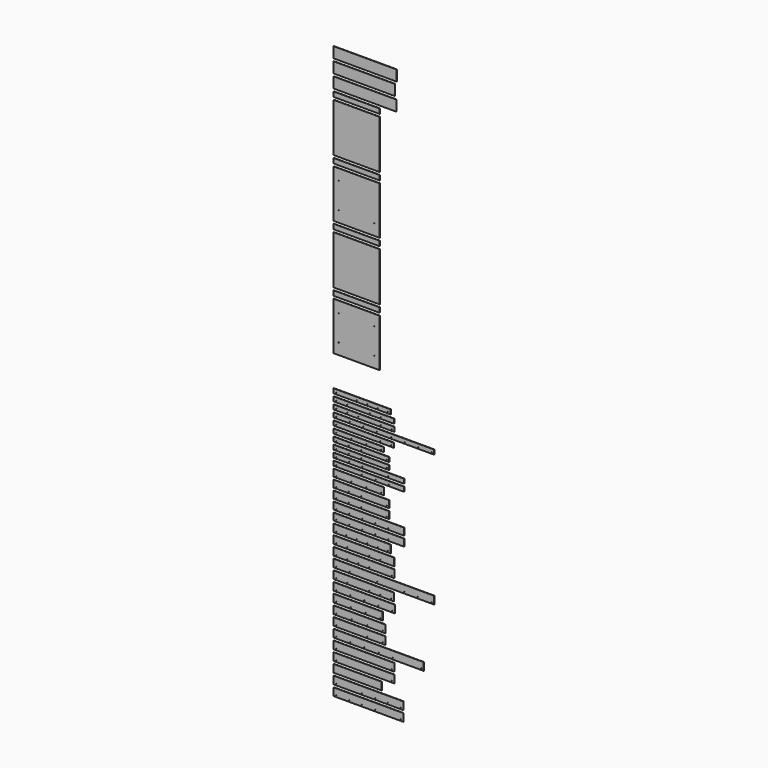
from build123d import *

# Parameters (mm, degrees)
F0_W     = 621.50625
F0_H     = 105.56875
F1_DEPTH = 3.175
F0_W_2   = 604.8375
F0_W_3   = 618.33125
F0_W_4   = 454.025
F0_H_2   = 47.625
F0_H_3   = 479.425
F0_H_4   = 473.075
F0_R     = 2.38125
F0_W_5   = 561.975
F0_H_5   = 76.2
F0_W_6   = 596.9
F0_W_7   = 598.4875
F0_W_8   = 992.1875
F0_W_9   = 595.3125
F0_W_10  = 484.1875
F0_W_11  = 511.175
F0_W_12  = 889
F0_W_13  = 600.075
F0_W_14  = 473.075
F0_W_15  = 688.975
F0_R_2   = 2.159
F0_H_6   = 44.45
F0_W_16  = 495.3
F0_W_17  = 547.6875
F0_W_18  = 695.325
F0_H_7   = 69.85


# Not quite as in the source:
# - a feature names something its author has since deleted; it is built from what else it names


with BuildPart() as f1:
    # F0 (on Front) → F1 (new body)
    with BuildSketch(Plane.XZ):
        with Locations((310.753125, -78.184375)):
            Rectangle(F0_W, F0_H)
    extrude(amount=F1_DEPTH)


with BuildPart() as f1b:
    # F0 (on Front) → F1, piece 2 (new body)
    with BuildSketch(Plane.XZ):
        with Locations((302.41875, -209.153125)):
            Rectangle(F0_W_2, F0_H)
    extrude(amount=F1_DEPTH)


with BuildPart() as f1c:
    # F0 (on Front) → F1, piece 3 (new body)
    with BuildSketch(Plane.XZ):
        with Locations((309.165625, -340.121875)):
            Rectangle(F0_W_3, F0_H)
    extrude(amount=F1_DEPTH)


with BuildPart() as f1d:
    # F0 (on Front) → F1, piece 4 (new body)
    with BuildSketch(Plane.XZ):
        with Locations((227.0125, -442.11875)):
            Rectangle(F0_W_4, F0_H_2)
    extrude(amount=F1_DEPTH)


with BuildPart() as f1e:
    # F0 (on Front) → F1, piece 5 (new body)
    with BuildSketch(Plane.XZ):
        with Locations((227.0125, -731.04375)):
            Rectangle(F0_W_4, F0_H_3)
    extrude(amount=F1_DEPTH)


with BuildPart() as f1f:
    # F0 (on Front) → F1, piece 6 (new body)
    with BuildSketch(Plane.XZ):
        with Locations((227.0125, -1019.96875)):
            Rectangle(F0_W_4, F0_H_2)
    extrude(amount=F1_DEPTH)


with BuildPart() as f1g:
    # F0 (on Front) → F1, piece 7 (new body)
    with BuildSketch(Plane.XZ):
        with Locations((227.0125, -1305.71875)):
            Rectangle(F0_W_4, F0_H_4)
        with Locations((50.8, -1432.71875)):
            Circle(F0_R, mode=Mode.SUBTRACT)
        with Locations((50.8, -1178.71875)):
            Circle(F0_R, mode=Mode.SUBTRACT)
        with Locations((403.225, -1432.71875)):
            Circle(F0_R, mode=Mode.SUBTRACT)
        with Locations((403.225, -1178.71875)):
            Circle(F0_R, mode=Mode.SUBTRACT)
    extrude(amount=F1_DEPTH)


with BuildPart() as f1h:
    # F0 (on Front) → F1, piece 8 (new body)
    with BuildSketch(Plane.XZ):
        with Locations((227.0125, -1591.46875)):
            Rectangle(F0_W_4, F0_H_2)
    extrude(amount=F1_DEPTH)


with BuildPart() as f1i:
    # F0 (on Front) → F1, piece 9 (new body)
    with BuildSketch(Plane.XZ):
        with Locations((227.0125, -1880.39375)):
            Rectangle(F0_W_4, F0_H_3)
    extrude(amount=F1_DEPTH)


with BuildPart() as f1j:
    # F0 (on Front) → F1, piece 10 (new body)
    with BuildSketch(Plane.XZ):
        with Locations((227.0125, -2169.31875)):
            Rectangle(F0_W_4, F0_H_2)
    extrude(amount=F1_DEPTH)


with BuildPart() as f1k:
    # F0 (on Front) → F1, piece 11 (new body)
    with BuildSketch(Plane.XZ):
        with Locations((227.0125, -2455.06875)):
            Rectangle(F0_W_4, F0_H_4)
        with Locations((50.8, -2582.06875)):
            Circle(F0_R, mode=Mode.SUBTRACT)
        with Locations((50.8, -2328.06875)):
            Circle(F0_R, mode=Mode.SUBTRACT)
        with Locations((403.225, -2582.06875)):
            Circle(F0_R, mode=Mode.SUBTRACT)
        with Locations((403.225, -2328.06875)):
            Circle(F0_R, mode=Mode.SUBTRACT)
    extrude(amount=F1_DEPTH)


with BuildPart() as f1l:
    # F0 (on Front) → F1, piece 12 (new body)
    with BuildSketch(Plane.XZ):
        with Locations((280.9875, -4209.25625)):
            Rectangle(F0_W_5, F0_H_5)
        with Locations((25.4, -4233.06875)):
            Circle(F0_R, mode=Mode.SUBTRACT)
        with Locations((127, -4233.06875)):
            Circle(F0_R, mode=Mode.SUBTRACT)
        with Locations((228.6, -4233.06875)):
            Circle(F0_R, mode=Mode.SUBTRACT)
        with Locations((333.375, -4233.06875)):
            Circle(F0_R, mode=Mode.SUBTRACT)
        with Locations((434.975, -4233.06875)):
            Circle(F0_R, mode=Mode.SUBTRACT)
        with Locations((536.575, -4233.06875)):
            Circle(F0_R, mode=Mode.SUBTRACT)
    extrude(amount=F1_DEPTH)


with BuildPart() as f1m:
    # F0 (on Front) → F1, piece 13 (new body)
    with BuildSketch(Plane.XZ):
        with Locations((298.45, -4310.85625)):
            Rectangle(F0_W_6, F0_H_5)
        with Locations((25.4, -4334.66875)):
            Circle(F0_R, mode=Mode.SUBTRACT)
        with Locations((134.9375, -4334.66875)):
            Circle(F0_R, mode=Mode.SUBTRACT)
        with Locations((244.475, -4334.66875)):
            Circle(F0_R, mode=Mode.SUBTRACT)
        with Locations((352.425, -4334.66875)):
            Circle(F0_R, mode=Mode.SUBTRACT)
        with Locations((461.9625, -4334.66875)):
            Circle(F0_R, mode=Mode.SUBTRACT)
        with Locations((571.5, -4334.66875)):
            Circle(F0_R, mode=Mode.SUBTRACT)
    extrude(amount=F1_DEPTH)


with BuildPart() as f1n:
    # F0 (on Front) → F1, piece 14 (new body)
    with BuildSketch(Plane.XZ):
        with Locations((299.24375, -4412.45625)):
            Rectangle(F0_W_7, F0_H_5)
        with Locations((25.4, -4436.26875)):
            Circle(F0_R, mode=Mode.SUBTRACT)
        with Locations((134.9375, -4436.26875)):
            Circle(F0_R, mode=Mode.SUBTRACT)
        with Locations((244.475, -4436.26875)):
            Circle(F0_R, mode=Mode.SUBTRACT)
        with Locations((354.0125, -4436.26875)):
            Circle(F0_R, mode=Mode.SUBTRACT)
        with Locations((463.55, -4436.26875)):
            Circle(F0_R, mode=Mode.SUBTRACT)
        with Locations((573.0875, -4436.26875)):
            Circle(F0_R, mode=Mode.SUBTRACT)
    extrude(amount=F1_DEPTH)


with BuildPart() as f1o:
    # F0 (on Front) → F1, piece 15 (new body)
    with BuildSketch(Plane.XZ):
        with Locations((496.09375, -4514.05625)):
            Rectangle(F0_W_8, F0_H_5)
        with Locations((25.4, -4537.86875)):
            Circle(F0_R, mode=Mode.SUBTRACT)
        with Locations((160.3375, -4537.86875)):
            Circle(F0_R, mode=Mode.SUBTRACT)
        with Locations((295.275, -4537.86875)):
            Circle(F0_R, mode=Mode.SUBTRACT)
        with Locations((430.2125, -4537.86875)):
            Circle(F0_R, mode=Mode.SUBTRACT)
        with Locations((561.975, -4537.86875)):
            Circle(F0_R, mode=Mode.SUBTRACT)
        with Locations((696.9125, -4537.86875)):
            Circle(F0_R, mode=Mode.SUBTRACT)
        with Locations((831.85, -4537.86875)):
            Circle(F0_R, mode=Mode.SUBTRACT)
        with Locations((966.7875, -4537.86875)):
            Circle(F0_R, mode=Mode.SUBTRACT)
    extrude(amount=F1_DEPTH)


with BuildPart() as f1p:
    # F0 (on Front) → F1, piece 16 (new body)
    with BuildSketch(Plane.XZ):
        with Locations((297.65625, -4615.65625)):
            Rectangle(F0_W_9, F0_H_5)
        with Locations((25.4, -4639.46875)):
            Circle(F0_R, mode=Mode.SUBTRACT)
        with Locations((133.35, -4639.46875)):
            Circle(F0_R, mode=Mode.SUBTRACT)
        with Locations((241.3, -4639.46875)):
            Circle(F0_R, mode=Mode.SUBTRACT)
        with Locations((354.0125, -4639.46875)):
            Circle(F0_R, mode=Mode.SUBTRACT)
        with Locations((461.9625, -4639.46875)):
            Circle(F0_R, mode=Mode.SUBTRACT)
        with Locations((569.9125, -4639.46875)):
            Circle(F0_R, mode=Mode.SUBTRACT)
    extrude(amount=F1_DEPTH)


with BuildPart() as f1q:
    # F0 (on Front) → F1, piece 17 (new body)
    with BuildSketch(Plane.XZ):
        with Locations((302.41875, -4717.25625)):
            Rectangle(F0_W_2, F0_H_5)
        with Locations((25.4, -4741.06875)):
            Circle(F0_R, mode=Mode.SUBTRACT)
        with Locations((163.5125, -4741.06875)):
            Circle(F0_R, mode=Mode.SUBTRACT)
        with Locations((302.41875, -4741.06875)):
            Circle(F0_R, mode=Mode.SUBTRACT)
        with Locations((441.325, -4741.06875)):
            Circle(F0_R, mode=Mode.SUBTRACT)
        with Locations((579.4375, -4741.06875)):
            Circle(F0_R, mode=Mode.SUBTRACT)
    extrude(amount=F1_DEPTH)


with BuildPart() as f1r:
    # F0 (on Front) → F1, piece 18 (new body)
    with BuildSketch(Plane.XZ):
        with Locations((242.09375, -4818.85625)):
            Rectangle(F0_W_10, F0_H_5)
        with Locations((25.4, -4842.66875)):
            Circle(F0_R, mode=Mode.SUBTRACT)
        with Locations((168.275, -4842.66875)):
            Circle(F0_R, mode=Mode.SUBTRACT)
        with Locations((315.9125, -4842.66875)):
            Circle(F0_R, mode=Mode.SUBTRACT)
        with Locations((458.7875, -4842.66875)):
            Circle(F0_R, mode=Mode.SUBTRACT)
    extrude(amount=F1_DEPTH)


with BuildPart() as f1s:
    # F0 (on Front) → F1, piece 19 (new body)
    with BuildSketch(Plane.XZ):
        with Locations((255.5875, -4920.45625)):
            Rectangle(F0_W_11, F0_H_5)
        with Locations((25.4, -4944.26875)):
            Circle(F0_R, mode=Mode.SUBTRACT)
        with Locations((177.8, -4944.26875)):
            Circle(F0_R, mode=Mode.SUBTRACT)
        with Locations((333.375, -4944.26875)):
            Circle(F0_R, mode=Mode.SUBTRACT)
        with Locations((485.775, -4944.26875)):
            Circle(F0_R, mode=Mode.SUBTRACT)
    extrude(amount=F1_DEPTH)


with BuildPart() as f1t:
    # F0 (on Front) → F1, piece 20 (new body)
    with BuildSketch(Plane.XZ):
        with Locations((255.5875, -5022.05625)):
            Rectangle(F0_W_11, F0_H_5)
        with Locations((25.4, -5045.86875)):
            Circle(F0_R, mode=Mode.SUBTRACT)
        with Locations((177.8, -5045.86875)):
            Circle(F0_R, mode=Mode.SUBTRACT)
        with Locations((333.375, -5045.86875)):
            Circle(F0_R, mode=Mode.SUBTRACT)
        with Locations((485.775, -5045.86875)):
            Circle(F0_R, mode=Mode.SUBTRACT)
    extrude(amount=F1_DEPTH)


with BuildPart() as f1u:
    # F0 (on Front) → F1, piece 21 (new body)
    with BuildSketch(Plane.XZ):
        with Locations((444.5, -5123.65625)):
            Rectangle(F0_W_12, F0_H_5)
        with Locations((25.4, -5147.46875)):
            Circle(F0_R, mode=Mode.SUBTRACT)
        with Locations((165.1, -5147.46875)):
            Circle(F0_R, mode=Mode.SUBTRACT)
        with Locations((304.8, -5147.46875)):
            Circle(F0_R, mode=Mode.SUBTRACT)
        with Locations((444.5, -5147.46875)):
            Circle(F0_R, mode=Mode.SUBTRACT)
        with Locations((584.2, -5147.46875)):
            Circle(F0_R, mode=Mode.SUBTRACT)
        with Locations((723.9, -5147.46875)):
            Circle(F0_R, mode=Mode.SUBTRACT)
        with Locations((863.6, -5147.46875)):
            Circle(F0_R, mode=Mode.SUBTRACT)
    extrude(amount=F1_DEPTH)


with BuildPart() as f1v:
    # F0 (on Front) → F1, piece 22 (new body)
    with BuildSketch(Plane.XZ):
        with Locations((300.0375, -5225.25625)):
            Rectangle(F0_W_13, F0_H_5)
        with Locations((25.4, -5249.06875)):
            Circle(F0_R, mode=Mode.SUBTRACT)
        with Locations((161.925, -5249.06875)):
            Circle(F0_R, mode=Mode.SUBTRACT)
        with Locations((300.0375, -5249.06875)):
            Circle(F0_R, mode=Mode.SUBTRACT)
        with Locations((438.15, -5249.06875)):
            Circle(F0_R, mode=Mode.SUBTRACT)
        with Locations((574.675, -5249.06875)):
            Circle(F0_R, mode=Mode.SUBTRACT)
    extrude(amount=F1_DEPTH)


with BuildPart() as f1w:
    # F0 (on Front) → F1, piece 23 (new body)
    with BuildSketch(Plane.XZ):
        with Locations((300.0375, -5326.85625)):
            Rectangle(F0_W_13, F0_H_5)
        with Locations((25.4, -5350.66875)):
            Circle(F0_R, mode=Mode.SUBTRACT)
        with Locations((161.925, -5350.66875)):
            Circle(F0_R, mode=Mode.SUBTRACT)
        with Locations((300.0375, -5350.66875)):
            Circle(F0_R, mode=Mode.SUBTRACT)
        with Locations((438.15, -5350.66875)):
            Circle(F0_R, mode=Mode.SUBTRACT)
        with Locations((574.675, -5350.66875)):
            Circle(F0_R, mode=Mode.SUBTRACT)
    extrude(amount=F1_DEPTH)


with BuildPart() as f1x:
    # F0 (on Front) → F1, piece 24 (new body)
    with BuildSketch(Plane.XZ):
        with Locations((236.5375, -5428.45625)):
            Rectangle(F0_W_14, F0_H_5)
    extrude(amount=F1_DEPTH)


with BuildPart() as f1y:
    # F0 (on Front) → F1, piece 25 (new body)
    with BuildSketch(Plane.XZ):
        with Locations((344.4875, -5530.05625)):
            Rectangle(F0_W_15, F0_H_5)
        with Locations((25.4, -5553.86875)):
            Circle(F0_R, mode=Mode.SUBTRACT)
        with Locations((152.4, -5553.86875)):
            Circle(F0_R, mode=Mode.SUBTRACT)
        with Locations((279.4, -5553.86875)):
            Circle(F0_R, mode=Mode.SUBTRACT)
        with Locations((409.575, -5553.86875)):
            Circle(F0_R, mode=Mode.SUBTRACT)
        with Locations((536.575, -5553.86875)):
            Circle(F0_R, mode=Mode.SUBTRACT)
        with Locations((663.575, -5553.86875)):
            Circle(F0_R, mode=Mode.SUBTRACT)
    extrude(amount=F1_DEPTH)


with BuildPart() as f1z:
    # F0 (on Front) → F1, piece 26 (new body)
    with BuildSketch(Plane.XZ):
        with Locations((344.4875, -5631.65625)):
            Rectangle(F0_W_15, F0_H_5)
        with Locations((25.4, -5655.46875)):
            Circle(F0_R_2, mode=Mode.SUBTRACT)
        with Locations((152.4, -5655.46875)):
            Circle(F0_R_2, mode=Mode.SUBTRACT)
        with Locations((279.4, -5655.46875)):
            Circle(F0_R_2, mode=Mode.SUBTRACT)
        with Locations((409.575, -5655.46875)):
            Circle(F0_R_2, mode=Mode.SUBTRACT)
        with Locations((536.575, -5655.46875)):
            Circle(F0_R_2, mode=Mode.SUBTRACT)
        with Locations((663.575, -5655.46875)):
            Circle(F0_R_2, mode=Mode.SUBTRACT)
    extrude(amount=F1_DEPTH)


with BuildPart() as f1ba:
    # F0 (on Front) → F1, piece 27 (new body)
    with BuildSketch(Plane.XZ):
        with Locations((280.9875, -3018.63125)):
            Rectangle(F0_W_5, F0_H_6)
        with Locations((25.4, -3026.56875)):
            Circle(F0_R, mode=Mode.SUBTRACT)
        with Locations((127, -3026.56875)):
            Circle(F0_R, mode=Mode.SUBTRACT)
        with Locations((228.6, -3026.56875)):
            Circle(F0_R, mode=Mode.SUBTRACT)
        with Locations((333.375, -3026.56875)):
            Circle(F0_R, mode=Mode.SUBTRACT)
        with Locations((434.975, -3026.56875)):
            Circle(F0_R, mode=Mode.SUBTRACT)
        with Locations((536.575, -3026.56875)):
            Circle(F0_R, mode=Mode.SUBTRACT)
    extrude(amount=F1_DEPTH)


with BuildPart() as f1bb:
    # F0 (on Front) → F1, piece 28 (new body)
    with BuildSketch(Plane.XZ):
        with Locations((298.45, -3088.48125)):
            Rectangle(F0_W_6, F0_H_6)
        with Locations((25.4, -3096.41875)):
            Circle(F0_R, mode=Mode.SUBTRACT)
        with Locations((133.35, -3096.41875)):
            Circle(F0_R, mode=Mode.SUBTRACT)
        with Locations((241.3, -3096.41875)):
            Circle(F0_R, mode=Mode.SUBTRACT)
        with Locations((355.6, -3096.41875)):
            Circle(F0_R, mode=Mode.SUBTRACT)
        with Locations((463.55, -3096.41875)):
            Circle(F0_R, mode=Mode.SUBTRACT)
        with Locations((571.5, -3096.41875)):
            Circle(F0_R, mode=Mode.SUBTRACT)
    extrude(amount=F1_DEPTH)


with BuildPart() as f1bc:
    # F0 (on Front) → F1, piece 29 (new body)
    with BuildSketch(Plane.XZ):
        with Locations((299.24375, -3158.33125)):
            Rectangle(F0_W_7, F0_H_6)
        with Locations((25.4, -3166.26875)):
            Circle(F0_R, mode=Mode.SUBTRACT)
        with Locations((134.9375, -3166.26875)):
            Circle(F0_R, mode=Mode.SUBTRACT)
        with Locations((244.475, -3166.26875)):
            Circle(F0_R, mode=Mode.SUBTRACT)
        with Locations((354.0125, -3166.26875)):
            Circle(F0_R, mode=Mode.SUBTRACT)
        with Locations((463.55, -3166.26875)):
            Circle(F0_R, mode=Mode.SUBTRACT)
        with Locations((573.0875, -3166.26875)):
            Circle(F0_R, mode=Mode.SUBTRACT)
    extrude(amount=F1_DEPTH)


with BuildPart() as f1bd:
    # F0 (on Front) → F1, piece 30 (new body)
    with BuildSketch(Plane.XZ):
        with Locations((496.09375, -3228.18125)):
            Rectangle(F0_W_8, F0_H_6)
        with Locations((25.4, -3236.11875)):
            Circle(F0_R, mode=Mode.SUBTRACT)
        with Locations((158.75, -3236.11875)):
            Circle(F0_R, mode=Mode.SUBTRACT)
        with Locations((292.1, -3236.11875)):
            Circle(F0_R, mode=Mode.SUBTRACT)
        with Locations((425.45, -3236.11875)):
            Circle(F0_R, mode=Mode.SUBTRACT)
        with Locations((566.7375, -3236.11875)):
            Circle(F0_R, mode=Mode.SUBTRACT)
        with Locations((700.0875, -3236.11875)):
            Circle(F0_R, mode=Mode.SUBTRACT)
        with Locations((833.4375, -3236.11875)):
            Circle(F0_R, mode=Mode.SUBTRACT)
        with Locations((966.7875, -3236.11875)):
            Circle(F0_R, mode=Mode.SUBTRACT)
    extrude(amount=F1_DEPTH)


with BuildPart() as f1be:
    # F0 (on Front) → F1, piece 31 (new body)
    with BuildSketch(Plane.XZ):
        with Locations((297.65625, -3298.03125)):
            Rectangle(F0_W_9, F0_H_6)
        with Locations((25.4, -3305.96875)):
            Circle(F0_R, mode=Mode.SUBTRACT)
        with Locations((133.35, -3305.96875)):
            Circle(F0_R, mode=Mode.SUBTRACT)
        with Locations((241.3, -3305.96875)):
            Circle(F0_R, mode=Mode.SUBTRACT)
        with Locations((354.0125, -3305.96875)):
            Circle(F0_R, mode=Mode.SUBTRACT)
        with Locations((461.9625, -3305.96875)):
            Circle(F0_R, mode=Mode.SUBTRACT)
        with Locations((569.9125, -3305.96875)):
            Circle(F0_R, mode=Mode.SUBTRACT)
    extrude(amount=F1_DEPTH)


with BuildPart() as f1bf:
    # F0 (on Front) → F1, piece 32 (new body)
    with BuildSketch(Plane.XZ):
        with Locations((247.65, -3367.88125)):
            Rectangle(F0_W_16, F0_H_6)
        with Locations((25.4, -3375.81875)):
            Circle(F0_R, mode=Mode.SUBTRACT)
        with Locations((173.0375, -3375.81875)):
            Circle(F0_R, mode=Mode.SUBTRACT)
        with Locations((322.2625, -3375.81875)):
            Circle(F0_R, mode=Mode.SUBTRACT)
        with Locations((469.9, -3375.81875)):
            Circle(F0_R, mode=Mode.SUBTRACT)
    extrude(amount=F1_DEPTH)


with BuildPart() as f1bg:
    # F0 (on Front) → F1, piece 33 (new body)
    with BuildSketch(Plane.XZ):
        with Locations((273.84375, -3437.73125)):
            Rectangle(F0_W_17, F0_H_6)
        with Locations((25.4, -3445.66875)):
            Circle(F0_R, mode=Mode.SUBTRACT)
        with Locations((149.225, -3445.66875)):
            Circle(F0_R, mode=Mode.SUBTRACT)
        with Locations((273.84375, -3445.66875)):
            Circle(F0_R, mode=Mode.SUBTRACT)
        with Locations((398.4625, -3445.66875)):
            Circle(F0_R, mode=Mode.SUBTRACT)
        with Locations((522.2875, -3445.66875)):
            Circle(F0_R, mode=Mode.SUBTRACT)
    extrude(amount=F1_DEPTH)


with BuildPart() as f1bh:
    # F0 (on Front) → F1, piece 34 (new body)
    with BuildSketch(Plane.XZ):
        with Locations((273.84375, -3507.58125)):
            Rectangle(F0_W_17, F0_H_6)
        with Locations((25.4, -3515.51875)):
            Circle(F0_R, mode=Mode.SUBTRACT)
        with Locations((149.225, -3515.51875)):
            Circle(F0_R, mode=Mode.SUBTRACT)
        with Locations((273.84375, -3515.51875)):
            Circle(F0_R, mode=Mode.SUBTRACT)
        with Locations((398.4625, -3515.51875)):
            Circle(F0_R, mode=Mode.SUBTRACT)
        with Locations((522.2875, -3515.51875)):
            Circle(F0_R, mode=Mode.SUBTRACT)
    extrude(amount=F1_DEPTH)


with BuildPart() as f1bi:
    # F0 (on Front) → F1, piece 35 (new body)
    with BuildSketch(Plane.XZ):
        with Locations((347.6625, -3577.43125)):
            Rectangle(F0_W_18, F0_H_6)
        with Locations((25.4, -3585.36875)):
            Circle(F0_R, mode=Mode.SUBTRACT)
        with Locations((153.9875, -3585.36875)):
            Circle(F0_R, mode=Mode.SUBTRACT)
        with Locations((282.575, -3585.36875)):
            Circle(F0_R, mode=Mode.SUBTRACT)
        with Locations((412.75, -3585.36875)):
            Circle(F0_R, mode=Mode.SUBTRACT)
        with Locations((541.3375, -3585.36875)):
            Circle(F0_R, mode=Mode.SUBTRACT)
        with Locations((669.925, -3585.36875)):
            Circle(F0_R, mode=Mode.SUBTRACT)
    extrude(amount=F1_DEPTH)


with BuildPart() as f1bj:
    # F0 (on Front) → F1, piece 36 (new body)
    with BuildSketch(Plane.XZ):
        with Locations((347.6625, -3647.28125)):
            Rectangle(F0_W_18, F0_H_6)
        with Locations((25.4, -3655.21875)):
            Circle(F0_R, mode=Mode.SUBTRACT)
        with Locations((152.4, -3655.21875)):
            Circle(F0_R, mode=Mode.SUBTRACT)
        with Locations((279.4, -3655.21875)):
            Circle(F0_R, mode=Mode.SUBTRACT)
        with Locations((415.925, -3655.21875)):
            Circle(F0_R, mode=Mode.SUBTRACT)
        with Locations((542.925, -3655.21875)):
            Circle(F0_R, mode=Mode.SUBTRACT)
        with Locations((669.925, -3655.21875)):
            Circle(F0_R, mode=Mode.SUBTRACT)
    extrude(amount=F1_DEPTH)


with BuildPart() as f1bk:
    # F0 (on Front) → F1, piece 37 (new body)
    with BuildSketch(Plane.XZ):
        with Locations((247.65, -3729.83125)):
            Rectangle(F0_W_16, F0_H_7)
        with Locations((25.4, -3750.46875)):
            Circle(F0_R, mode=Mode.SUBTRACT)
        with Locations((173.0375, -3750.46875)):
            Circle(F0_R, mode=Mode.SUBTRACT)
        with Locations((322.2625, -3750.46875)):
            Circle(F0_R, mode=Mode.SUBTRACT)
        with Locations((469.9, -3750.46875)):
            Circle(F0_R, mode=Mode.SUBTRACT)
    extrude(amount=F1_DEPTH)


with BuildPart() as f1bl:
    # F0 (on Front) → F1, piece 38 (new body)
    with BuildSketch(Plane.XZ):
        with Locations((273.84375, -3825.08125)):
            Rectangle(F0_W_17, F0_H_7)
        with Locations((25.4, -3845.71875)):
            Circle(F0_R, mode=Mode.SUBTRACT)
        with Locations((149.225, -3845.71875)):
            Circle(F0_R, mode=Mode.SUBTRACT)
        with Locations((273.84375, -3845.71875)):
            Circle(F0_R, mode=Mode.SUBTRACT)
        with Locations((398.4625, -3845.71875)):
            Circle(F0_R, mode=Mode.SUBTRACT)
        with Locations((522.2875, -3845.71875)):
            Circle(F0_R, mode=Mode.SUBTRACT)
    extrude(amount=F1_DEPTH)


with BuildPart() as f1bm:
    # F0 (on Front) → F1, piece 39 (new body)
    with BuildSketch(Plane.XZ):
        with Locations((273.84375, -3920.33125)):
            Rectangle(F0_W_17, F0_H_7)
        with Locations((25.4, -3940.96875)):
            Circle(F0_R, mode=Mode.SUBTRACT)
        with Locations((149.225, -3940.96875)):
            Circle(F0_R, mode=Mode.SUBTRACT)
        with Locations((273.84375, -3940.96875)):
            Circle(F0_R, mode=Mode.SUBTRACT)
        with Locations((398.4625, -3940.96875)):
            Circle(F0_R, mode=Mode.SUBTRACT)
        with Locations((522.2875, -3940.96875)):
            Circle(F0_R, mode=Mode.SUBTRACT)
    extrude(amount=F1_DEPTH)


with BuildPart() as f1bn:
    # F0 (on Front) → F1, piece 40 (new body)
    with BuildSketch(Plane.XZ):
        with Locations((347.6625, -4015.58125)):
            Rectangle(F0_W_18, F0_H_7)
        with Locations((25.4, -4036.21875)):
            Circle(F0_R, mode=Mode.SUBTRACT)
        with Locations((153.9875, -4036.21875)):
            Circle(F0_R, mode=Mode.SUBTRACT)
        with Locations((282.575, -4036.21875)):
            Circle(F0_R, mode=Mode.SUBTRACT)
        with Locations((412.75, -4036.21875)):
            Circle(F0_R, mode=Mode.SUBTRACT)
        with Locations((541.3375, -4036.21875)):
            Circle(F0_R, mode=Mode.SUBTRACT)
        with Locations((669.925, -4036.21875)):
            Circle(F0_R, mode=Mode.SUBTRACT)
    extrude(amount=F1_DEPTH)


with BuildPart() as f1bo:
    # F0 (on Front) → F1, piece 41 (new body)
    with BuildSketch(Plane.XZ):
        with Locations((347.6625, -4110.83125)):
            Rectangle(F0_W_18, F0_H_7)
        with Locations((25.4, -4131.46875)):
            Circle(F0_R, mode=Mode.SUBTRACT)
        with Locations((153.9875, -4131.46875)):
            Circle(F0_R, mode=Mode.SUBTRACT)
        with Locations((282.575, -4131.46875)):
            Circle(F0_R, mode=Mode.SUBTRACT)
        with Locations((412.75, -4131.46875)):
            Circle(F0_R, mode=Mode.SUBTRACT)
        with Locations((541.3375, -4131.46875)):
            Circle(F0_R, mode=Mode.SUBTRACT)
        with Locations((669.925, -4131.46875)):
            Circle(F0_R, mode=Mode.SUBTRACT)
    extrude(amount=F1_DEPTH)


solid = Compound([f1.part, f1b.part, f1c.part, f1d.part, f1e.part, f1f.part, f1g.part, f1h.part, f1i.part, f1j.part, f1k.part, f1l.part, f1m.part, f1n.part, f1o.part, f1p.part, f1q.part, f1r.part, f1s.part, f1t.part, f1u.part, f1v.part, f1w.part, f1x.part, f1y.part, f1z.part, f1ba.part, f1bb.part, f1bc.part, f1bd.part, f1be.part, f1bf.part, f1bg.part, f1bh.part, f1bi.part, f1bj.part, f1bk.part, f1bl.part, f1bm.part, f1bn.part, f1bo.part])
